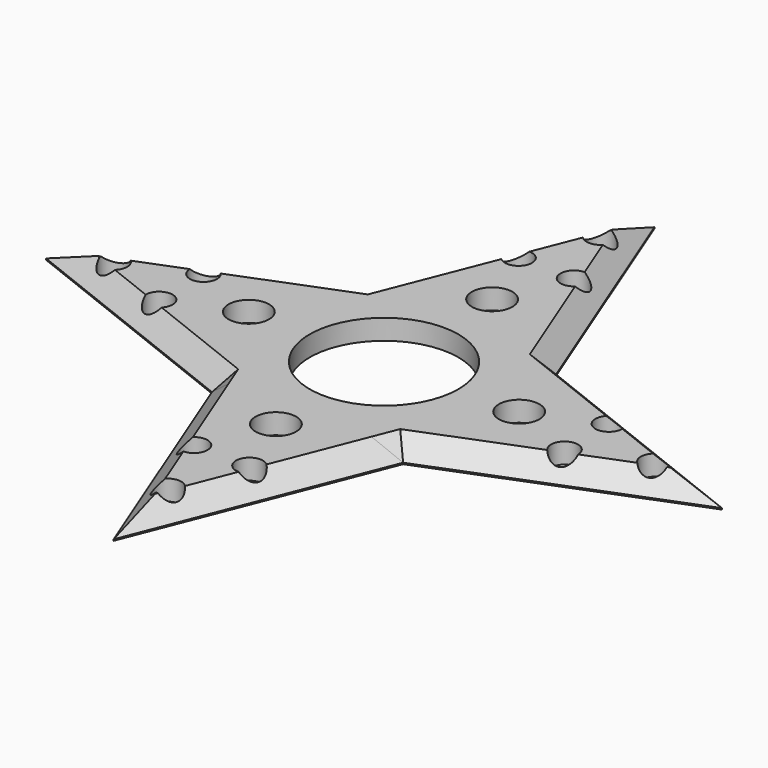
from build123d import *

# Parameters (mm, degrees)
F0_R         = 2
F0_R_2       = 3
F0_R_3       = 11
F1_DEPTH     = 3
F2_T4_DEPTH  = 52.9473251324
F3_T4_DEPTH  = 48.8454257103
F4_T4_DEPTH  = 56.77883553
F4_T10_DEPTH = 56.77883553
F4_T15_DEPTH = 52.9473251324
F4_T20_DEPTH = 52.9473251324
F4_T25_DEPTH = 56.77883553
F4_T31_DEPTH = 56.77883553
F4_T36_DEPTH = 52.9473251324
F4_T41_DEPTH = 52.9473251324
F4_T47_DEPTH = 52.9473251324
F4_T51_DEPTH = 52.9473251324
F4_T58_DEPTH = 52.9473251324
F4_T62_DEPTH = 52.9473251324


# Not quite as in the source:
# - a fillet or chamfer that OpenCascade refuses, or shapes differently, is made with other operations: its cross-section is extruded or revolved along the edge and cut away or added


with BuildPart() as f1:
    # F0 (on Top) → F1 (new body)
    with BuildSketch(Plane.XY):
        Polygon((-14.1421356237, 14.1421356237), (-50, 0), (-14.1421356237, -14.1421356237), (0, -50), (14.1421356237, -14.1421356237), (50, 0), (14.1421356237, 14.1421356237), (0, 50), align=None)
        with Locations((-4.1164257564, -30)):
            Circle(F0_R, mode=Mode.SUBTRACT)
        with Locations((-30, -4.0949434042)):
            Circle(F0_R, mode=Mode.SUBTRACT)
        with Locations((0, -40)):
            Circle(F0_R, mode=Mode.SUBTRACT)
        with Locations((4.0949434042, -30)):
            Circle(F0_R, mode=Mode.SUBTRACT)
        with Locations((0, -20)):
            Circle(F0_R_2, mode=Mode.SUBTRACT)
        with Locations((30, -4.1164257564)):
            Circle(F0_R, mode=Mode.SUBTRACT)
        with Locations((-40, 0)):
            Circle(F0_R, mode=Mode.SUBTRACT)
        with Locations((-30, 4.1164257564)):
            Circle(F0_R, mode=Mode.SUBTRACT)
        with Locations((-20, 0)):
            Circle(F0_R_2, mode=Mode.SUBTRACT)
        with Locations((-4.0949434042, 30)):
            Circle(F0_R, mode=Mode.SUBTRACT)
        Circle(F0_R_3, mode=Mode.SUBTRACT)
        with Locations((20, 0)):
            Circle(F0_R_2, mode=Mode.SUBTRACT)
        with Locations((0, 20)):
            Circle(F0_R_2, mode=Mode.SUBTRACT)
        with Locations((30, 4.0949434042)):
            Circle(F0_R, mode=Mode.SUBTRACT)
        with Locations((40, 0)):
            Circle(F0_R, mode=Mode.SUBTRACT)
        with Locations((4.1164257564, 30)):
            Circle(F0_R, mode=Mode.SUBTRACT)
        with Locations((0, 40)):
            Circle(F0_R, mode=Mode.SUBTRACT)
    extrude(amount=F1_DEPTH)

    # F2: chamfer of 2.8 on 1 edges, made by hand


with BuildPart() as f2_tool2:
    # F2_s3 → F2_t4 (new body)
    with BuildSketch(Plane(origin=(-19.7071398503, -49.9681212794, 0), x_dir=(0, 0, 1), z_dir=(0.3668907842, 0.930264023, 0))):
        Polygon((0.2, 18.3445392079), (3, 15.5445392079), (3, 18.3445392079), align=None)
    extrude(amount=F2_T4_DEPTH)

    split(bisect_by=Plane(origin=(6.730442375, -17.0652648437, 0), x_dir=(0, 0, 1), z_dir=(0.3668907842, -0.930264023, 0)), keep=Keep.TOP)


with BuildPart() as f1_1:
    add(f1.part)

    # F2_t1: cut F2_tool2
    add(f2_tool2.part, mode=Mode.SUBTRACT)

    # F3: chamfer of 2.8 on 1 edges, made by hand


with BuildPart() as f3_tool2:
    # F3_s3 → F3_t4 (new body)
    with BuildSketch(Plane(origin=(0.2812542134, -0.7131295943, 0), x_dir=(0, 0, 1), z_dir=(0.3668907842, -0.930264023, 0))):
        Polygon((3, 15.5445392079), (0.2, 18.3445392079), (3, 18.3445392079), align=None)
    extrude(amount=F3_T4_DEPTH)

    split(bisect_by=Plane(origin=(-6.730442375, -17.0652648437, 0), x_dir=(0, 0, 1), z_dir=(-0.3668907842, -0.930264023, 0)), keep=Keep.TOP)


with BuildPart() as f1_2:
    add(f1_1.part)

    # F3_t1: cut F3_tool2
    add(f3_tool2.part, mode=Mode.SUBTRACT)

    # F4: chamfer of 2.8 on 6 edges, made by hand


with BuildPart() as f4_tool2:
    # F4_s3 → F4_t4 (new body)
    with BuildSketch(Plane(origin=(-2.8511866823, -1.1244916409, 0), x_dir=(0, 0, 1), z_dir=(0.930264023, 0.3668907842, 0))):
        Polygon((3, 15.5445392079), (0.2, 18.3445392079), (3, 18.3445392079), align=None)
    extrude(amount=F4_T4_DEPTH)

    split(bisect_by=Plane(origin=(17.0652648437, -6.730442375, 0), x_dir=(0, 0, 1), z_dir=(-0.930264023, 0.3668907842, 0)), keep=Keep.TOP)

    split(bisect_by=Plane(origin=(8.6256588242, -3.4019102659, 9.272269604), x_dir=(0.3668907842, 0.930264023, 0), z_dir=(0.657795999, -0.2594309614, 0.7071067812)), keep=Keep.TOP)


with BuildPart() as f1_3:
    add(f1_2.part)

    # F4_t1: cut F4_tool2
    add(f4_tool2.part, mode=Mode.SUBTRACT)


with BuildPart() as f4_tool8:
    # F4_s9 → F4_t10 (new body)
    with BuildSketch(Plane(origin=(-2.8511866823, -1.1244916409, 0), x_dir=(0, 0, 1), z_dir=(0.930264023, 0.3668907842, 0))):
        Polygon((3, 15.5445392079), (0.2, 18.3445392079), (3, 18.3445392079), align=None)
    extrude(amount=F4_T10_DEPTH)

    split(bisect_by=Plane(origin=(17.0652648437, -6.730442375, 0), x_dir=(0, 0, 1), z_dir=(0.930264023, -0.3668907842, 0)), keep=Keep.TOP)


with BuildPart() as f1_4:
    add(f1_3.part)

    # F4_t7: cut F4_tool8
    add(f4_tool8.part, mode=Mode.SUBTRACT)


with BuildPart() as f4_tool13:
    # F4_s14 → F4_t15 (new body)
    with BuildSketch(Plane(origin=(49.9681212794, -19.7071398503, 0), x_dir=(0, 0, 1), z_dir=(-0.930264023, 0.3668907842, 0))):
        Polygon((3, 15.5445392079), (0.2, 18.3445392079), (3, 18.3445392079), align=None)
    extrude(amount=F4_T15_DEPTH)

    split(bisect_by=Plane(origin=(17.0652648437, 6.730442375, 0), x_dir=(0, 0, 1), z_dir=(0.930264023, 0.3668907842, 0)), keep=Keep.TOP)


with BuildPart() as f1_5:
    add(f1_4.part)

    # F4_t12: cut F4_tool13
    add(f4_tool13.part, mode=Mode.SUBTRACT)


with BuildPart() as f4_tool18:
    # F4_s19 → F4_t20 (new body)
    with BuildSketch(Plane(origin=(-0.2812542134, 0.7131295943, 0), x_dir=(0, 0, 1), z_dir=(-0.3668907842, 0.930264023, 0))):
        Polygon((3, 15.5445392079), (0.2, 18.3445392079), (3, 18.3445392079), align=None)
    extrude(amount=F4_T20_DEPTH)

    split(bisect_by=Plane(origin=(6.730442375, 17.0652648437, 0), x_dir=(0, 0, 1), z_dir=(0.3668907842, 0.930264023, 0)), keep=Keep.TOP)


with BuildPart() as f1_6:
    add(f1_5.part)

    # F4_t17: cut F4_tool18
    add(f4_tool18.part, mode=Mode.SUBTRACT)


with BuildPart() as f4_tool23:
    # F4_s24 → F4_t25 (new body)
    with BuildSketch(Plane(origin=(2.8511866823, -1.1244916409, 0), x_dir=(0, 0, 1), z_dir=(-0.930264023, 0.3668907842, 0))):
        Polygon((3, -15.5445392079), (0.2, -18.3445392079), (3, -18.3445392079), align=None)
    extrude(amount=F4_T25_DEPTH)

    split(bisect_by=Plane(origin=(-17.0652648437, -6.730442375, 0), x_dir=(0, 0, 1), z_dir=(0.930264023, 0.3668907842, 0)), keep=Keep.TOP)

    split(bisect_by=Plane(origin=(-8.6256588242, -3.4019102659, 9.272269604), x_dir=(0.3668907842, -0.930264023, 0), z_dir=(-0.657795999, -0.2594309614, 0.7071067812)), keep=Keep.TOP)


with BuildPart() as f1_7:
    add(f1_6.part)

    # F4_t22: cut F4_tool23
    add(f4_tool23.part, mode=Mode.SUBTRACT)


with BuildPart() as f4_tool29:
    # F4_s30 → F4_t31 (new body)
    with BuildSketch(Plane(origin=(2.8511866823, -1.1244916409, 0), x_dir=(0, 0, 1), z_dir=(-0.930264023, 0.3668907842, 0))):
        Polygon((3, -15.5445392079), (0.2, -18.3445392079), (3, -18.3445392079), align=None)
    extrude(amount=F4_T31_DEPTH)

    split(bisect_by=Plane(origin=(-17.0652648437, -6.730442375, 0), x_dir=(0, 0, 1), z_dir=(-0.930264023, -0.3668907842, 0)), keep=Keep.TOP)


with BuildPart() as f1_8:
    add(f1_7.part)

    # F4_t28: cut F4_tool29
    add(f4_tool29.part, mode=Mode.SUBTRACT)


with BuildPart() as f4_tool34:
    # F4_s35 → F4_t36 (new body)
    with BuildSketch(Plane(origin=(-0.7131295943, -0.2812542134, 0), x_dir=(0, 0, 1), z_dir=(-0.930264023, -0.3668907842, 0))):
        Polygon((0.2, 18.3445392079), (3, 15.5445392079), (3, 18.3445392079), align=None)
    extrude(amount=F4_T36_DEPTH)

    split(bisect_by=Plane(origin=(-17.0652648437, 6.730442375, 0), x_dir=(0, 0, 1), z_dir=(-0.930264023, 0.3668907842, 0)), keep=Keep.TOP)


with BuildPart() as f1_9:
    add(f1_8.part)

    # F4_t33: cut F4_tool34
    add(f4_tool34.part, mode=Mode.SUBTRACT)


with BuildPart() as f4_tool39:
    # F4_s40 → F4_t41 (new body)
    with BuildSketch(Plane(origin=(19.7071398503, 49.9681212794, 0), x_dir=(0, 0, 1), z_dir=(-0.3668907842, -0.930264023, 0))):
        Polygon((3, 15.5445392079), (0.2, 18.3445392079), (3, 18.3445392079), align=None)
    extrude(amount=F4_T41_DEPTH)

    split(bisect_by=Plane(origin=(-6.730442375, 17.0652648437, 0), x_dir=(0, 0, 1), z_dir=(-0.3668907842, 0.930264023, 0)), keep=Keep.TOP)


with BuildPart() as f1_10:
    add(f1_9.part)

    # F4_t38: cut F4_tool39
    add(f4_tool39.part, mode=Mode.SUBTRACT)


with BuildPart() as f4_tool45:
    # F4_s46 → F4_t47 (new body)
    with BuildSketch(Plane(origin=(-0.2812542134, 0.7131295943, 0), x_dir=(0, 0, 1), z_dir=(-0.3668907842, 0.930264023, 0))):
        Polygon((3, 15.5445392079), (0.2, 18.3445392079), (3, 18.3445392079), align=None)
    extrude(amount=F4_T47_DEPTH)

    split(bisect_by=Plane(origin=(6.730442375, 17.0652648437, 0), x_dir=(0, 0, 1), z_dir=(-0.3668907842, -0.930264023, 0)), keep=Keep.TOP)


with BuildPart() as f4_tool49:
    # F4_s50 → F4_t51 (new body)
    with BuildSketch(Plane(origin=(49.9681212794, -19.7071398503, 0), x_dir=(0, 0, 1), z_dir=(-0.930264023, 0.3668907842, 0))):
        Polygon((3, 15.5445392079), (0.2, 18.3445392079), (3, 18.3445392079), align=None)
    extrude(amount=F4_T51_DEPTH)

    split(bisect_by=Plane(origin=(17.0652648437, 6.730442375, 0), x_dir=(0, 0, 1), z_dir=(-0.930264023, -0.3668907842, 0)), keep=Keep.TOP)


with BuildPart() as f4_tool45_1:
    add(f4_tool45.part)

    # F4_t53: intersect F4_tool49
    add(f4_tool49.part, mode=Mode.INTERSECT)


with BuildPart() as f1_11:
    add(f1_10.part)

    # F4_t43: cut F4_tool45
    add(f4_tool45_1.part, mode=Mode.SUBTRACT)


with BuildPart() as f4_tool56:
    # F4_s57 → F4_t58 (new body)
    with BuildSketch(Plane(origin=(-0.7131295943, -0.2812542134, 0), x_dir=(0, 0, 1), z_dir=(-0.930264023, -0.3668907842, 0))):
        Polygon((0.2, 18.3445392079), (3, 15.5445392079), (3, 18.3445392079), align=None)
    extrude(amount=F4_T58_DEPTH)

    split(bisect_by=Plane(origin=(-17.0652648437, 6.730442375, 0), x_dir=(0, 0, 1), z_dir=(0.930264023, -0.3668907842, 0)), keep=Keep.TOP)


with BuildPart() as f4_tool60:
    # F4_s61 → F4_t62 (new body)
    with BuildSketch(Plane(origin=(19.7071398503, 49.9681212794, 0), x_dir=(0, 0, 1), z_dir=(-0.3668907842, -0.930264023, 0))):
        Polygon((3, 15.5445392079), (0.2, 18.3445392079), (3, 18.3445392079), align=None)
    extrude(amount=F4_T62_DEPTH)

    split(bisect_by=Plane(origin=(-6.730442375, 17.0652648437, 0), x_dir=(0, 0, 1), z_dir=(0.3668907842, -0.930264023, 0)), keep=Keep.TOP)


with BuildPart() as f4_tool56_1:
    add(f4_tool56.part)

    # F4_t64: intersect F4_tool60
    add(f4_tool60.part, mode=Mode.INTERSECT)


with BuildPart() as f1_12:
    add(f1_11.part)

    # F4_t54: cut F4_tool56
    add(f4_tool56_1.part, mode=Mode.SUBTRACT)


solid = f1_12.part
